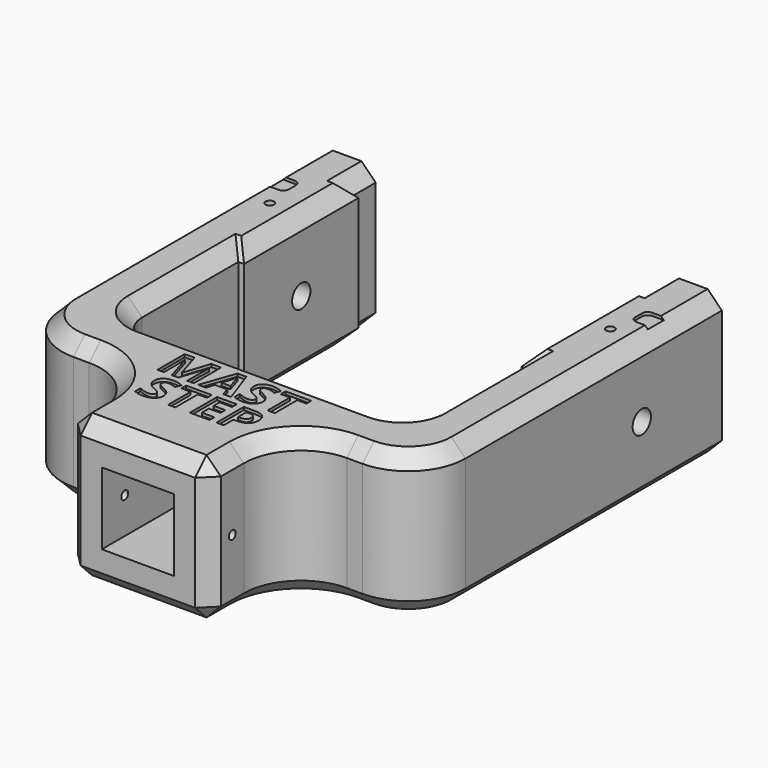
from build123d import *

# Parameters (mm, degrees)
F1_DEPTH      = 25
F1_DEPTH_BACK = 25
F2_W          = 25.2
F2_H          = 25.2
F3_DEPTH      = 40
F4_R          = 4
F5_DEPTH      = 141.001
F6_SIZE       = 5
F7_R          = 1.5
F8_DEPTH      = 50.001
F9_R          = 1.5
F10_DEPTH     = 95.5010001
F11_TEXT_SIZE = 16.6666666667
F12_DEPTH     = 1
F13_R         = 4.05
F14_DEPTH     = 20


# Not quite as in the source:
# - Text() gives the source's letters only with a copy of the font that has no kerning and outlines rounded to 1/6400 em; it was checked with that copy


with BuildPart() as f1:
    # F0 (on Top) → F1 (new body, two sides)
    with BuildSketch(Plane.XY) as f1_sk:
        with BuildLine():
            Line((0, 0), (25, 0))
            Line((25, 0), (25, 15))
            ThreePointArc((25, 15), (30.8578643763, 29.1421356237), (45, 35))
            Line((45, 35), (50.5, 35))
            ThreePointArc((50.5, 35), (64.6421356237, 40.8578643763), (70.5, 55))
            Line((70.5, 55), (70.5, 157))
            Line((70.5, 157), (70.5, 167))
            Line((70.5, 167), (50.5, 167))
            Line((50.5, 167), (50.5, 157))
            Line((50.5, 157), (48.5, 157))
            Line((48.5, 157), (48.5, 107))
            Line((48.5, 107), (50.5, 107))
            Line((50.5, 107), (50.5, 65))
            ThreePointArc((50.5, 65), (47.5710678119, 57.9289321881), (40.5, 55))
            Line((40.5, 55), (0, 55))
            Line((0, 55), (-40.5, 55))
            ThreePointArc((-40.5, 55), (-47.5710678119, 57.9289321881), (-50.5, 65))
            Line((-50.5, 65), (-50.5, 107))
            Line((-50.5, 107), (-48.5, 107))
            Line((-48.5, 107), (-48.5, 157))
            Line((-48.5, 157), (-50.5, 157))
            Line((-50.5, 157), (-50.5, 167))
            Line((-50.5, 167), (-70.5, 167))
            Line((-70.5, 167), (-70.5, 157))
            Line((-70.5, 157), (-70.5, 55))
            ThreePointArc((-70.5, 55), (-64.6421356237, 40.8578643763), (-50.5, 35))
            Line((-50.5, 35), (-45, 35))
            ThreePointArc((-45, 35), (-30.8578643763, 29.1421356237), (-25, 15))
            Line((-25, 15), (-25, 0))
            Line((-25, 0), (0, 0))
        make_face()
    extrude(amount=F1_DEPTH)
    extrude(f1_sk.sketch, amount=-F1_DEPTH_BACK)

    # F2 (on face) → F3 (cut)
    with BuildSketch(Plane.XZ):
        Rectangle(F2_W, F2_H)
    extrude(amount=-F3_DEPTH, mode=Mode.SUBTRACT)

    # F4 (on face) → F5 (cut, through all)
    with BuildSketch(Plane(origin=(-70.5, 0, 0), x_dir=(0, -1, 0), z_dir=(-1, 0, 0))):
        with Locations((-132, 0)):
            Circle(F4_R)
    extrude(amount=-F5_DEPTH, mode=Mode.SUBTRACT)

    # F6
    f6_edges = [f1.edges().sort_by_distance(p)[0] for p in [
        (25, 0, 0),
        (-25, 0, 0),
        (-30.857864, 29.142136, 25),
        (-25, 7.5, 25),
        (-47.75, 35, 25),
        (-64.642136, 40.857864, 25),
        (-70.5, 111, 25),
        (-50.5, 86, 25),
        (-48.5, 132, 25),
        (-50.5, 162, 25),
        (-47.571068, 57.928932, 25),
        (0, 55, 25),
        (47.571068, 57.928932, 25),
        (50.5, 86, 25),
        (48.5, 132, 25),
        (50.5, 162, 25),
        (70.5, 111, 25),
        (64.642136, 40.857864, 25),
        (30.857864, 29.142136, 25),
        (47.75, 35, 25),
        (25, 7.5, 25),
        (0, 0, 25),
        (49.5, 107, 25),
        (49.5, 157, 25),
        (-49.5, 157, 25),
        (-49.5, 107, 25),
        (70.5, 111, -25),
        (50.5, 86, -25),
        (48.5, 132, -25),
        (50.5, 162, -25),
        (49.5, 157, -25),
        (49.5, 107, -25),
        (47.571068, 57.928932, -25),
        (0, 55, -25),
        (-47.571068, 57.928932, -25),
        (-50.5, 86, -25),
        (-49.5, 107, -25),
        (-48.5, 132, -25),
        (-49.5, 157, -25),
        (-50.5, 162, -25),
        (64.642136, 40.857864, -25),
        (47.75, 35, -25),
        (30.857864, 29.142136, -25),
        (25, 7.5, -25),
        (0, 0, -25),
        (-25, 7.5, -25),
        (-30.857864, 29.142136, -25),
        (-47.75, 35, -25),
        (-64.642136, 40.857864, -25),
        (-70.5, 111, -25),
    ]]
    chamfer(f6_edges, length=F6_SIZE)

    # F7 (on face) → F8 (cut, through all)
    with BuildSketch(Plane.XY.offset(25)):
        with Locations((-59.5, 132)):
            Circle(F7_R)
        with Locations((59.5, 132)):
            Circle(F7_R)
    extrude(amount=-F8_DEPTH, mode=Mode.SUBTRACT)

    # F9 (on face) → F10 (cut, through all)
    with BuildSketch(Plane(origin=(-25, 0, 0), x_dir=(0, -1, 0), z_dir=(-1, 0, 0))):
        with Locations((-10, 0)):
            Circle(F9_R)
    extrude(amount=-F10_DEPTH, mode=Mode.SUBTRACT)

    # F11 (on face) → F12 (cut)
    with BuildSketch(Plane.XY.offset(25)):
        with BuildLine():
            Line((70.5, 146.6229859591), (62.5, 146.6229859591))
            ThreePointArc((62.5, 146.6229859591), (61.0857864376, 146.0371995214), (60.5, 144.6229859591))
            Line((60.5, 144.6229859591), (60.5, 141.6229859591))
            ThreePointArc((60.5, 141.6229859591), (61.0857864376, 140.2087723967), (62.5, 139.6229859591))
            Line((62.5, 139.6229859591), (70.5, 139.6229859591))
            Line((70.5, 139.6229859591), (70.5, 146.6229859591))
        make_face()
        with BuildLine():
            Line((-60.5, 141.6229859591), (-60.5, 144.6229859591))
            ThreePointArc((-60.5, 144.6229859591), (-61.0857864376, 146.0371995214), (-62.5, 146.6229859591))
            Line((-62.5, 146.6229859591), (-70.5, 146.6229859591))
            Line((-70.5, 146.6229859591), (-70.5, 139.6229859591))
            Line((-70.5, 139.6229859591), (-62.5, 139.6229859591))
            ThreePointArc((-62.5, 139.6229859591), (-61.0857864376, 140.2087723967), (-60.5, 141.6229859591))
        make_face()
        with Locations((-23.3958333333, 35.9334971694)):
            Text('MAST', F11_TEXT_SIZE, font='Open Sans', font_style=FontStyle.BOLD, text_align=(TextAlign.LEFT, TextAlign.BOTTOM))
        with Locations((-19.48046875, 21.6453020573)):
            Text('STEP', F11_TEXT_SIZE, font='Open Sans', font_style=FontStyle.BOLD, text_align=(TextAlign.LEFT, TextAlign.BOTTOM))
    extrude(amount=-F12_DEPTH, mode=Mode.SUBTRACT)

    # F13 (on face) → F14 (cut)
    with BuildSketch(Plane(origin=(0, 167, 0), x_dir=(-1, 0, 0), z_dir=(0, 1, 0))):
        with Locations((60.5, -10)):
            Circle(F13_R)
        with Locations((60.5, 10)):
            Circle(F13_R)
        with Locations((-60.5, -10)):
            Circle(F13_R)
        with Locations((-60.5, 10)):
            Circle(F13_R)
    extrude(amount=-F14_DEPTH, mode=Mode.SUBTRACT)


solid = f1.part
